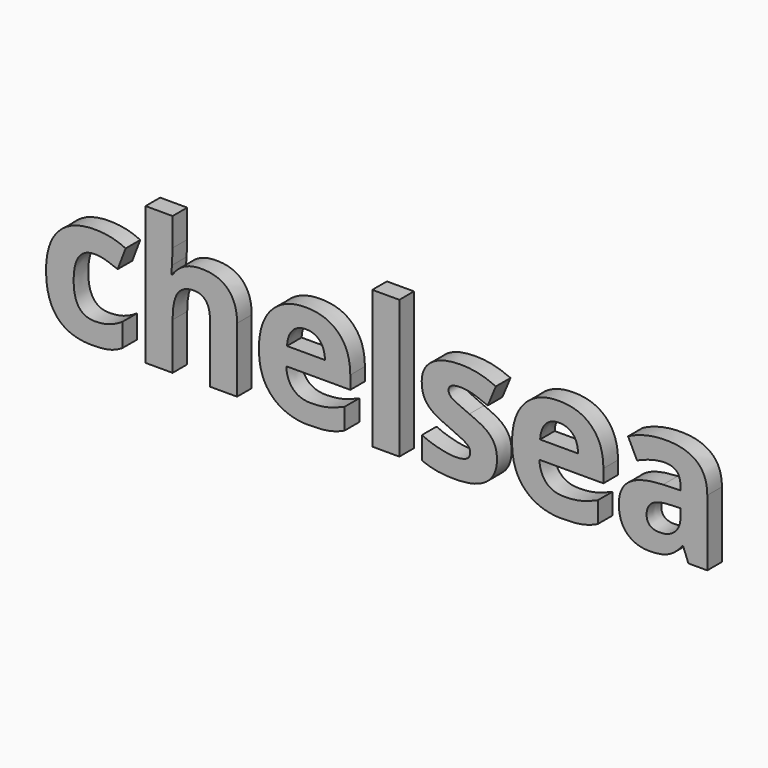
from build123d import *

# Parameters (mm, degrees)
F0_TEXT_SIZE = 63.0766670737
F1_DEPTH     = 6.35


# Not quite as in the source:
# - Text() gives the source's letters only with a copy of the font that has no kerning and outlines rounded to 1/6400 em; it was checked with that copy


with BuildPart() as f1:
    # F0 (on Front) → F1 (new body)
    with BuildSketch(Plane.XZ):
        with Locations((-116.7384143919, -20.5739997327)):
            Text('chelsea', F0_TEXT_SIZE, font='Open Sans', font_style=FontStyle.BOLD, text_align=(TextAlign.LEFT, TextAlign.BOTTOM))
    extrude(amount=F1_DEPTH)


solid = f1.part
